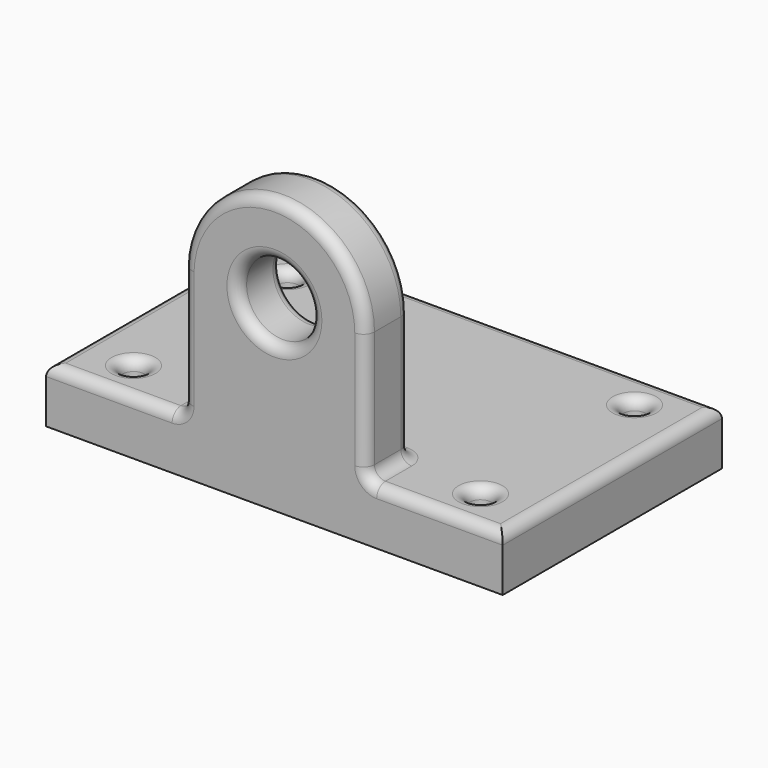
from build123d import *

# Parameters (mm, degrees)
F0_W     = 125
F0_H     = 75
F1_DEPTH = 15
F3_R     = 10
F4_DEPTH = 15
F5_R     = 3
F6_DEPTH = 25
F7_R     = 3


with BuildPart() as f1:
    # F0 (on Top) → F1 (new body)
    with BuildSketch(Plane.XY):
        Rectangle(F0_W, F0_H)
    extrude(amount=F1_DEPTH)

    # F3 (on face) → F4 (join)
    with BuildSketch(Plane.XZ.offset(37.5)):
        with BuildLine():
            Line((25, 15), (25, 50))
            ThreePointArc((25, 50), (0.2580876326, 25.00133222), (-24.9946712619, 49.4838522411))
            Line((-24.9946712619, 49.4838522411), (-24.9946712619, 15))
            Line((-24.9946712619, 15), (25, 15))
        make_face()
        with BuildLine():
            ThreePointArc((-24.9946712619, 49.4838522411), (0.2580876326, 25.00133222), (25, 50))
            ThreePointArc((25, 50), (0.2580876326, 74.99866778), (-24.9946712619, 50.5161477589))
            Line((-24.9946712619, 50.5161477589), (-24.9946712619, 49.4838522411))
        make_face()
        with Locations((0, 50)):
            Circle(F3_R, mode=Mode.SUBTRACT)
    extrude(amount=-F4_DEPTH)

    # F5 (on face) → F6 (cut)
    with BuildSketch(Plane.XY.offset(15)):
        with Locations((-47.5, 26.3456302691)):
            Circle(F5_R)
        with Locations((47.5, 26.3456302691)):
            Circle(F5_R)
        with Locations((47.5, -26.3456302691)):
            Circle(F5_R)
        with Locations((-47.5, -26.3456302691)):
            Circle(F5_R)
    extrude(amount=-F6_DEPTH, mode=Mode.SUBTRACT)

    # F7
    f7_edges = [f1.edges().sort_by_distance(p)[0] for p in [
        (43.75, -37.5, 15),
        (25, -30, 15),
        (62.5, 0, 15),
        (0.002664, -22.5, 15),
        (0, 37.5, 15),
        (-24.994671, -30, 15),
        (-62.5, 0, 15),
        (-43.747336, -37.5, 15),
        (-50.5, -26.34563, 15),
        (44.5, -26.34563, 15),
        (-50.5, 26.34563, 15),
        (44.5, 26.34563, 15),
        (25, -22.5, 32.5),
        (0.258088, -22.5, 74.998668),
        (-24.994671, -22.5, 32.758074),
        (-10, -22.5, 50),
        (-10, -37.5, 50),
        (-24.994671, -37.5, 32.758074),
        (0.258088, -37.5, 74.998668),
        (25, -37.5, 32.5),
    ]]
    fillet(f7_edges, radius=F7_R)


solid = f1.part
